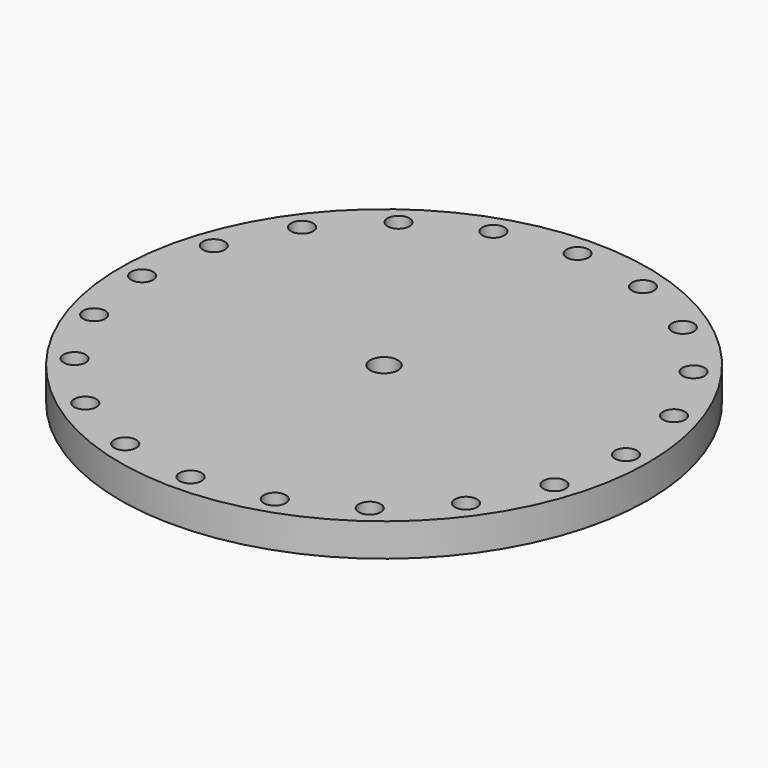
from build123d import *

# Parameters (mm, degrees)
F0_R            = 76.2
F0_R_2          = 4
F1_DEPTH        = 9.525
F3_D            = 6.35
F3_COPIES_COUNT = 20


# Not quite as in the source:
# - a pattern or mirror of a feature is missing from the dataset's text; its kind, count and spacing are read off the source's solid


with BuildPart() as f1:
    # F0 (on Top) → F1 (new body)
    with BuildSketch(Plane.XY):
        Circle(F0_R)
        Circle(F0_R_2, mode=Mode.SUBTRACT)
    extrude(amount=F1_DEPTH)

    # F3 (through all)
    with Locations(Plane.XY.offset(9.525)):
        with Locations((0, 69.85)):
            f3 = Hole(F3_D / 2)

    # F3_copies: F3 ×20 about axis
    f3_copies_axis = Axis((0, 0, 0), (0, 0, 1))
    for i in range(1, F3_COPIES_COUNT):
        add(f3.rotate(f3_copies_axis, i * 360 / F3_COPIES_COUNT), mode=Mode.SUBTRACT)


solid = f1.part
